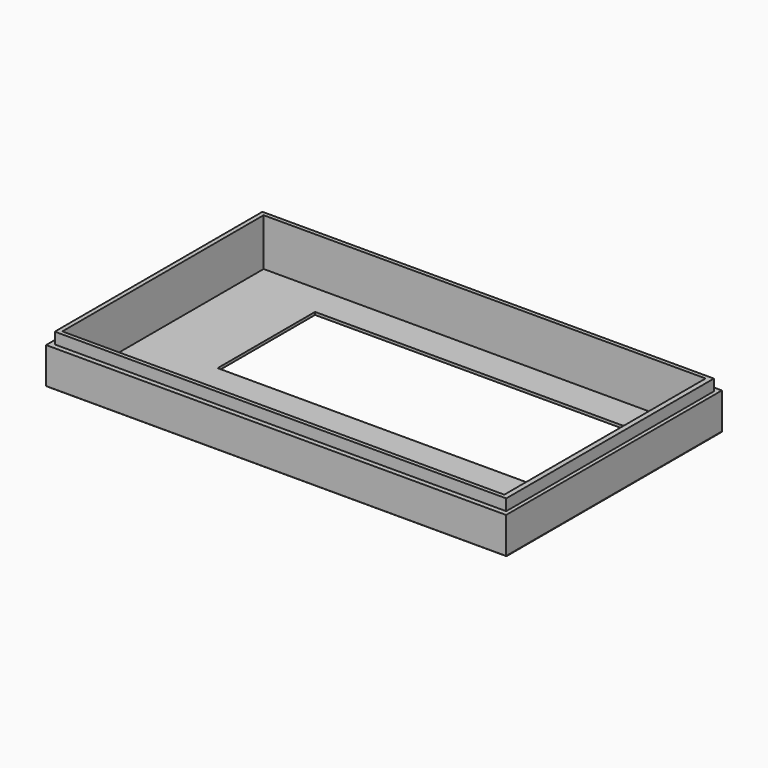
from build123d import *

# Parameters (mm, degrees)
F0_W        = 102
F0_H        = 59.8
F0_W_2      = 98
F0_H_2      = 55.8
F1_DEPTH    = 8
F2_W        = 102.0620055497
F2_H        = 59.6651937813
F3_DEPTH    = 0.6
F4_W        = 100.1025550067
F4_H        = 57.5502440333
F4_W_2      = 98
F4_H_2      = 55.8
F5_DEPTH    = 2.5
F6_T1_DEPTH = 105.5349790349
F6_T3_DEPTH = 3.6684549434
F6_T5_DEPTH = 66.8066222098
F6_T7_DEPTH = 3.6684549117
F6_T9_DEPTH = 105.5349790665
F7_W        = 73
F7_H        = 27
F8_DEPTH    = 8.6010001


# Not quite as in the source:
# - a fillet or chamfer that OpenCascade refuses, or shapes differently, is made with other operations: its cross-section is extruded or revolved along the edge and cut away or added


with BuildPart() as f1:
    # F0 (on Top) → F1 (new body)
    with BuildSketch(Plane.XY):
        with Locations((-11.1629452705, -1.3489569187)):
            Rectangle(F0_W, F0_H)
        with Locations((-11.1629452705, -1.3489569187)):
            Rectangle(F0_W_2, F0_H_2, mode=Mode.SUBTRACT)
    extrude(amount=F1_DEPTH)

    # F2 (on Top) → F3 (join)
    with BuildSketch(Plane.XY):
        with Locations((-11.096207425, -1.3842275366)):
            Rectangle(F2_W, F2_H)
    extrude(amount=-F3_DEPTH)

    # F4 (on face) → F5 (join)
    with BuildSketch(Plane.XY.offset(8)):
        with Locations((-11.0803488642, -1.3563353568)):
            Rectangle(F4_W, F4_H)
        with Locations((-11.1629452705, -1.3489569187)):
            Rectangle(F4_W_2, F4_H_2, mode=Mode.SUBTRACT)
    extrude(amount=F5_DEPTH)

    # F6: fillet of radius 2 on 4 edges, made by hand

    # F6_s2 → F6_t1 (cut)
    with BuildSketch(Plane.YZ.offset(-65.6979244141)):
        with BuildLine():
            ThreePointArc((-29.7885387415, -0.6), (-30.5631354108, -0.4439088915), (-31.2168244272, 0))
            Line((-31.2168244272, 0), (-31.2168244272, -0.6))
            Line((-31.2168244272, -0.6), (-29.7885387415, -0.6))
        make_face()
    extrude(amount=F6_T1_DEPTH, mode=Mode.SUBTRACT)

    # F6_s4 → F6_t3 (cut)
    with BuildSketch(Plane.YZ.offset(39.8370546207)):
        with BuildLine():
            ThreePointArc((-29.7885387415, -0.6), (-30.5631354108, -0.4439088915), (-31.2168244272, 0))
            Line((-31.2168244272, 0), (-31.2168244272, -0.6))
            Line((-31.2168244272, -0.6), (-29.7885387415, -0.6))
        make_face()
    extrude(amount=F6_T3_DEPTH, mode=Mode.SUBTRACT)

    # F6_s6 → F6_t5 (cut)
    with BuildSketch(Plane.XZ.offset(-32.0190835683)):
        with BuildLine():
            ThreePointArc((-60.6989245141, -0.6), (-61.4735211834, -0.4439088915), (-62.1272101998, 0))
            Line((-62.1272101998, 0), (-62.1272101998, -0.6))
            Line((-62.1272101998, -0.6), (-60.6989245141, -0.6))
        make_face()
        with BuildLine():
            ThreePointArc((38.5065096641, -0.6), (39.2811063334, -0.4439088915), (39.9347953498, 0))
            Line((39.9347953498, 0), (39.9347953498, -0.6))
            Line((39.9347953498, -0.6), (38.5065096641, -0.6))
        make_face()
    extrude(amount=F6_T5_DEPTH, mode=Mode.SUBTRACT)

    # F6_s8 → F6_t7 (cut)
    with BuildSketch(Plane.YZ.offset(39.8370546524)):
        with BuildLine():
            ThreePointArc((28.448369354, 0), (27.7946803375, -0.4439088915), (27.0200836683, -0.6))
            Line((27.0200836683, -0.6), (28.448369354, -0.6))
            Line((28.448369354, -0.6), (28.448369354, 0))
        make_face()
    extrude(amount=F6_T7_DEPTH, mode=Mode.SUBTRACT)

    # F6_s10 → F6_t9 (cut)
    with BuildSketch(Plane.YZ.offset(-65.6979244141)):
        with BuildLine():
            ThreePointArc((28.448369354, 0), (27.7946803375, -0.4439088915), (27.0200836683, -0.6))
            Line((27.0200836683, -0.6), (28.448369354, -0.6))
            Line((28.448369354, -0.6), (28.448369354, 0))
        make_face()
    extrude(amount=F6_T9_DEPTH, mode=Mode.SUBTRACT)

    # F7 (on face) → F8 (cut, through all)
    with BuildSketch(Plane.XY.offset(8)):
        with Locations((-6.6629452705, 6.0510430813)):
            Rectangle(F7_W, F7_H)
    extrude(amount=-F8_DEPTH, mode=Mode.SUBTRACT)


solid = f1.part
